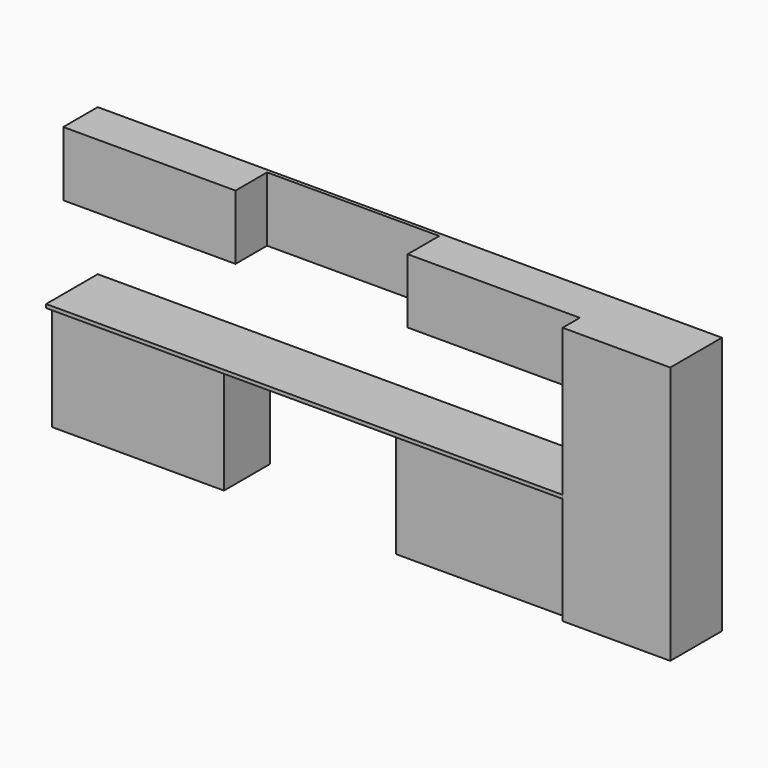
from build123d import *

# Parameters (mm, degrees)
F0_W     = 609.6
F0_H     = 762
F1_DEPTH = 406.4
F2_DEPTH = 457.2
F0_H_2   = 457.2
F3_DEPTH = 304.8
F4_W     = 1219.2
F4_H     = 406.4
F5_DEPTH = 25.4
F6_DEPTH = 25.4


with BuildPart() as f1:
    # F0 (on Front) → F1 (new body)
    with BuildSketch(Plane.XZ):
        with Locations((609.6, 0)):
            Rectangle(F0_W, F0_H)
        with Locations((1219.2, 0)):
            Rectangle(F0_W, F0_H)
    extrude(amount=F1_DEPTH)

    # F0 (on Front) → F2 (join)
    with BuildSketch(Plane.XZ):
        Polygon((1524, 381), (1524, -381), (2286, -381), (2286, 1447.8), (1524, 1447.8), (1524, 990.6), align=None)
    extrude(amount=F2_DEPTH)

    # F0 (on Front) → F3, piece 2 (join)
    with BuildSketch(Plane.XZ):
        with Locations((609.6, 1219.2)):
            Rectangle(F0_W, F0_H_2)
        with Locations((1219.2, 1219.2)):
            Rectangle(F0_W, F0_H_2)
    extrude(amount=F3_DEPTH)



with BuildPart() as f1b:
    # F0 (on Front) → F1, piece 2 (new body)
    with BuildSketch(Plane.XZ):
        with Locations((-1828.8, 0)):
            Rectangle(F0_W, F0_H)
        with Locations((-1219.2, 0)):
            Rectangle(F0_W, F0_H)
    extrude(amount=F1_DEPTH)


with BuildPart() as f3:
    # F0 (on Front) → F3 (new body)
    with BuildSketch(Plane.XZ):
        with Locations((-1219.2, 1219.2)):
            Rectangle(F0_W, F0_H_2)
        with Locations((-1828.8, 1219.2)):
            Rectangle(F0_W, F0_H_2)
    extrude(amount=F3_DEPTH)


with BuildPart() as f1_1:
    add(f1.part)

    add(f1b.part)  # F5 merges F1b
    # F4 (on face) → F5 (join)
    with BuildSketch(Plane.XY.offset(381)):
        Polygon((1523.5787630081, -457.2), (1523.5787630081, 0), (-914.4, 0), (-914.4, -406.4), (-2133.6, -406.4), (-2133.6, -457.2), align=None)
        with Locations((-1524, -203.2)):
            Rectangle(F4_W, F4_H)
    extrude(amount=F5_DEPTH)


    add(f3.part)  # F6 merges F3
    # F0 (on Front) → F6 (join)
    with BuildSketch(Plane.XZ):
        with Locations((0, 1219.2)):
            Rectangle(F0_W, F0_H_2)
        with Locations((-609.6, 1219.2)):
            Rectangle(F0_W, F0_H_2)
    extrude(amount=F6_DEPTH)


solid = f1_1.part
